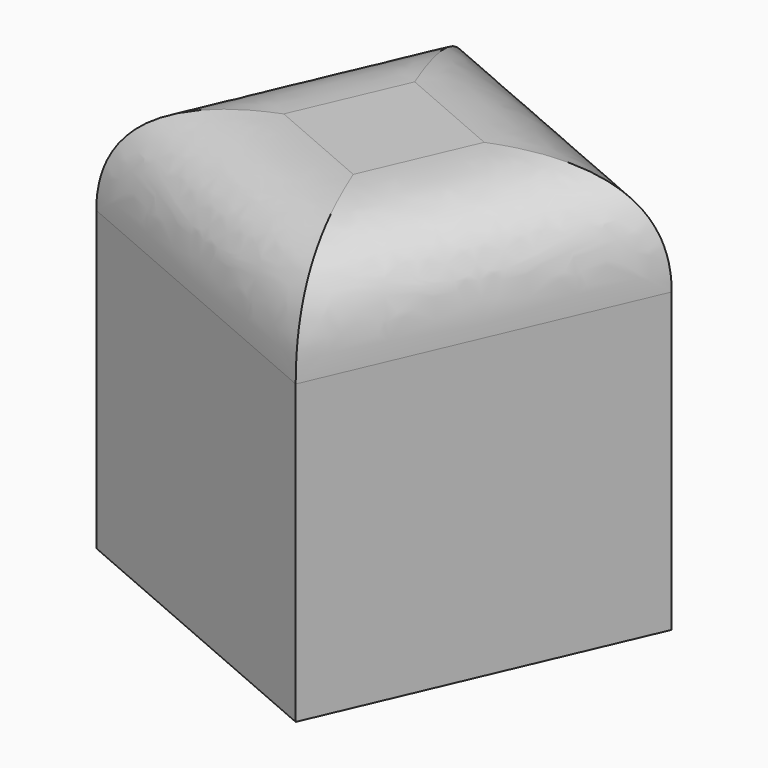
from build123d import *

# Parameters (mm, degrees)
F1_DEPTH    = 74.93201
F2_T1_DEPTH = 161.3731420762
F2_T3_DEPTH = 161.3731420762
F2_T5_DEPTH = 161.3731420762
F2_T7_DEPTH = 161.3731420762


# Not quite as in the source:
# - a fillet or chamfer that OpenCascade refuses, or shapes differently, is made with other operations: its cross-section is extruded or revolved along the edge and cut away or added


with BuildPart() as f1:
    # F0 (on Top) → F1 (new body)
    with BuildSketch(Plane.XY):
        Polygon((-56.1133213341, -3.1524337828), (-31.7345000803, 53.1710572541), (-88.0579911172, 77.5498785079), (-112.436812371, 21.226387471), align=None)
    extrude(amount=F1_DEPTH)

    # F2: fillet of radius 20 on 4 edges, made by hand

    # F2_s2 → F2_t1 (cut)
    with BuildSketch(Plane(origin=(-29.8642383226, -68.9966976654, 0), x_dir=(0, 0, 1), z_dir=(0.3972229615, 0.917722136, 0))):
        with BuildLine():
            add(Edge.make_bspline(
                [(54.93201, -50.2442180275), (74.93201, -50.2442180275), (74.93201, -70.2442180275)],
                knots=[0, 0, 0, 1, 1, 1], degree=2, weights=[1, 1, 1]))
            Line((74.93201, -70.2442180275), (74.93201, -50.2442180275))
            Line((74.93201, -50.2442180275), (54.93201, -50.2442180275))
        make_face()
    extrude(amount=F2_T1_DEPTH, mode=Mode.SUBTRACT)

    # F2_s4 → F2_t3 (cut)
    with BuildSketch(Plane(origin=(-0.2241242898, 0.0970090081, 0), x_dir=(0, 0, 1), z_dir=(-0.917722136, 0.3972229615, 0))):
        with BuildLine():
            add(Edge.make_bspline(
                [(54.93201, 36.1905841301), (74.93201, 36.1905841301), (74.93201, 16.1905841301)],
                knots=[0, 0, 0, 1, 1, 1], degree=2, weights=[1, 1, 1]))
            Line((74.93201, 16.1905841301), (74.93201, 36.1905841301))
            Line((74.93201, 36.1905841301), (54.93201, 36.1905841301))
        make_face()
    extrude(amount=F2_T3_DEPTH, mode=Mode.SUBTRACT)

    # F2_s6 → F2_t5 (cut)
    with BuildSketch(Plane(origin=(34.236879084, 79.0990069677, 0), x_dir=(0, 0, 1), z_dir=(-0.3972229615, -0.917722136, 0))):
        with BuildLine():
            add(Edge.make_bspline(
                [(54.93201, 111.6173601037), (74.93201, 111.6173601037), (74.93201, 91.6173601037)],
                knots=[0, 0, 0, 1, 1, 1], degree=2, weights=[1, 1, 1]))
            Line((74.93201, 91.6173601037), (74.93201, 111.6173601037))
            Line((74.93201, 111.6173601037), (54.93201, 111.6173601037))
        make_face()
    extrude(amount=F2_T5_DEPTH, mode=Mode.SUBTRACT)

    # F2_s8 → F2_t7 (cut)
    with BuildSketch(Plane(origin=(-148.3198289229, 64.1981264147, 0), x_dir=(0, 0, 1), z_dir=(0.917722136, -0.3972229615, 0))):
        with BuildLine():
            add(Edge.make_bspline(
                [(54.93201, 25.1825579461), (74.93201, 25.1825579461), (74.93201, 5.1825579461)],
                knots=[0, 0, 0, 1, 1, 1], degree=2, weights=[1, 1, 1]))
            Line((74.93201, 5.1825579461), (74.93201, 25.1825579461))
            Line((74.93201, 25.1825579461), (54.93201, 25.1825579461))
        make_face()
    extrude(amount=F2_T7_DEPTH, mode=Mode.SUBTRACT)


solid = f1.part
